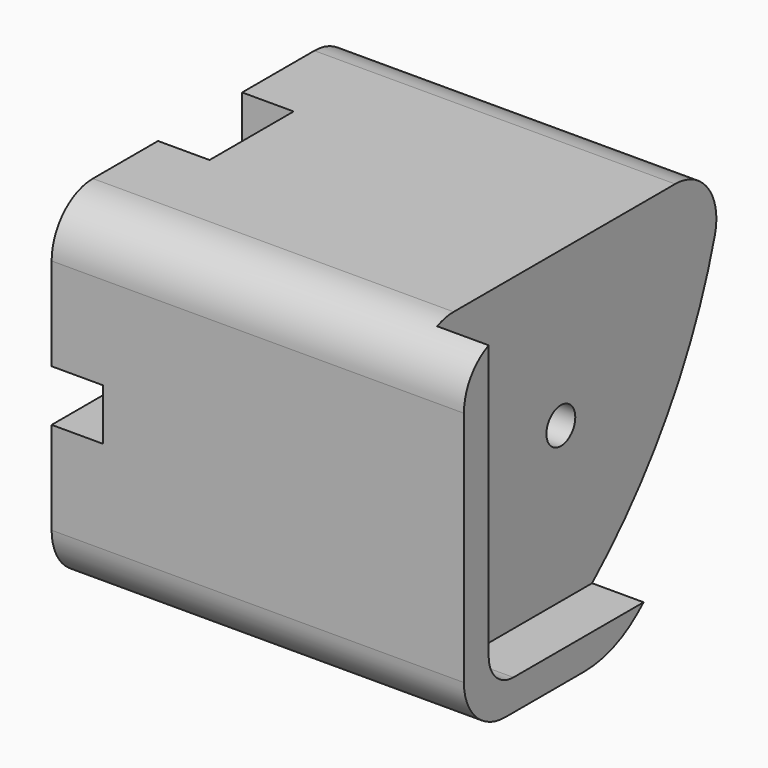
from build123d import *

# Parameters (mm, degrees)
F1_DEPTH     = 5
F0_R         = 1.75
F2_DEPTH     = 20
F3_R         = 3.25
F4_DEPTH     = 15
F5_R         = 1.35
F5_W         = 2.6
F5_H         = 6
F5_W_2       = 5
F6_DEPTH     = 5
F7_DEPTH     = 10
F8_R         = 3
F9_R         = 5
F10_T1_DEPTH = 14.8533585862
F11_R        = 1
F12_R        = 5
F13_R        = 5
F14_R        = 10


# Not quite as in the source:
# - a fillet or chamfer that OpenCascade refuses, or shapes differently, is made with other operations: its cross-section is extruded or revolved along the edge and cut away or added


with BuildPart() as f1:
    # F0 (on Right) → F1 (new body)
    with BuildSketch(Plane.YZ):
        Polygon((-15, -15), (-15, 0), (-15, 15), (-18, 15), (-18, 0), (-18, -18), (0, -18), (0, -15), align=None)
        with BuildLine():
            Line((3.7889535467, -15), (0, -15))
            Line((0, -15), (0, -18))
            ThreePointArc((0, -18), (1.9315685392, -16.546846326), (3.7889535467, -15))
        make_face()
    extrude(amount=F1_DEPTH)

    # F0 (on Right) → F2 (join)
    with BuildSketch(Plane.YZ):
        with BuildLine():
            Line((-15, 15), (-15, 0))
            Line((-15, 0), (-15, -15))
            Line((-15, -15), (0, -15))
            Line((0, -15), (3.7889535467, -15))
            ThreePointArc((3.7889535467, -15), (14.5947925758, -1.4591648304), (20, 15))
            Line((20, 15), (-15, 15))
        make_face()
        Circle(F0_R, mode=Mode.SUBTRACT)
        Polygon((-15, -15), (-15, 0), (-15, 15), (-18, 15), (-18, 0), (-18, -18), (0, -18), (0, -15), align=None)
        with BuildLine():
            Line((3.7889535467, -15), (0, -15))
            Line((0, -15), (0, -18))
            ThreePointArc((0, -18), (1.9315685392, -16.546846326), (3.7889535467, -15))
        make_face()
    extrude(amount=-F2_DEPTH)

    # F3 (on face) → F4 (join)
    with BuildSketch(Plane(origin=(-20, 0, 0), x_dir=(0, -1, 0), z_dir=(-1, 0, 0))):
        with BuildLine():
            Line((18, -18), (18, 15))
            Line((18, 15), (-20, 15))
            ThreePointArc((-20, 15), (-13.3934629181, -3.5566441928), (0, -18))
            Line((0, -18), (18, -18))
        make_face()
        Circle(F3_R, mode=Mode.SUBTRACT)
    extrude(amount=F4_DEPTH)

    # F5 (on face) → F6 (cut)
    with BuildSketch(Plane(origin=(-35, 0, 0), x_dir=(0, -1, 0), z_dir=(-1, 0, 0))):
        with Locations((-10.5, 12)):
            Circle(F5_R)
        with Locations((10.5, 12)):
            Circle(F5_R)
        with Locations((3.8, 12)):
            Rectangle(F5_W, F5_H)
        with BuildLine():
            Line((2.5, 2.0766559657), (2.5, 9))
            Line((2.5, 9), (-2.5, 9))
            Line((-2.5, 9), (-2.5, 2.0766559657))
            ThreePointArc((-2.5, 2.0766559657), (0, 3.25), (2.5, 2.0766559657))
        make_face()
        with Locations((0, 12)):
            Rectangle(F5_W_2, F5_H)
        with Locations((-3.8, 12)):
            Rectangle(F5_W, F5_H)
        with BuildLine():
            Line((18, 1), (3.0923292192, 1))
            ThreePointArc((3.0923292192, 1), (3.2103403217, 0.5061768651), (3.25, 0))
            ThreePointArc((3.25, 0), (3.0567548152, -1.1039701083), (2.5, -2.0766559657))
            Line((2.5, -2.0766559657), (2.5, -4))
            Line((2.5, -4), (18, -4))
            Line((18, -4), (18, 1))
        make_face()
        with BuildLine():
            ThreePointArc((2.5, -2.0766559657), (0, -3.25), (-2.5, -2.0766559657))
            Line((-2.5, -2.0766559657), (-2.5, -4))
            Line((-2.5, -4), (0, -4))
            Line((0, -4), (2.5, -4))
            Line((2.5, -4), (2.5, -2.0766559657))
        make_face()
    extrude(amount=-F6_DEPTH, mode=Mode.SUBTRACT)

    # F7 (cut): faces of the model
    f7_faces = [f1.faces().sort_by_distance(p)[0] for p in [
        (-30, 10.5, 12),
        (-30, -10.5, 12),
    ]]
    extrude(f7_faces, amount=-F7_DEPTH, mode=Mode.SUBTRACT)

    # F8
    f8_edges = [f1.edges().sort_by_distance(p)[0] for p in [
        (2.5, -15, -15),
    ]]
    fillet(f8_edges, radius=F8_R)

    # F9
    f9_edges = [f1.edges().sort_by_distance(p)[0] for p in [
        (-15, -18, -18),
    ]]
    fillet(f9_edges, radius=F9_R)

    # F10: fillet of radius 5 on 1 edges, made by hand

    # F10_s2 → F10_t1 (join)
    with BuildSketch(Plane.YZ.offset(-35)):
        with BuildLine():
            ThreePointArc((-1.4413434345, -4), (0.7514538853, -3.4935108673), (2.5, -2.0766559657))
            Line((2.5, -2.0766559657), (2.5, -4))
            Line((2.5, -4), (-1.4413434345, -4))
        make_face()
    extrude(amount=F10_T1_DEPTH)

    # F11
    f11_edges = [f1.edges().sort_by_distance(p)[0] for p in [
        (-32.5, 2.5, 9),
        (-32.5, -2.5, 9),
    ]]
    fillet(f11_edges, radius=F11_R)

    # F12
    f12_edges = [f1.edges().sort_by_distance(p)[0] for p in [
        (-17.5, 20, 15),
    ]]
    fillet(f12_edges, radius=F12_R)

    # F13
    f13_edges = [f1.edges().sort_by_distance(p)[0] for p in [
        (-15, -18, 15),
    ]]
    fillet(f13_edges, radius=F13_R)

    # F14
    f14_edges = [f1.edges().sort_by_distance(p)[0] for p in [
        (-15, 0, -18),
    ]]
    fillet(f14_edges, radius=F14_R)


solid = f1.part
